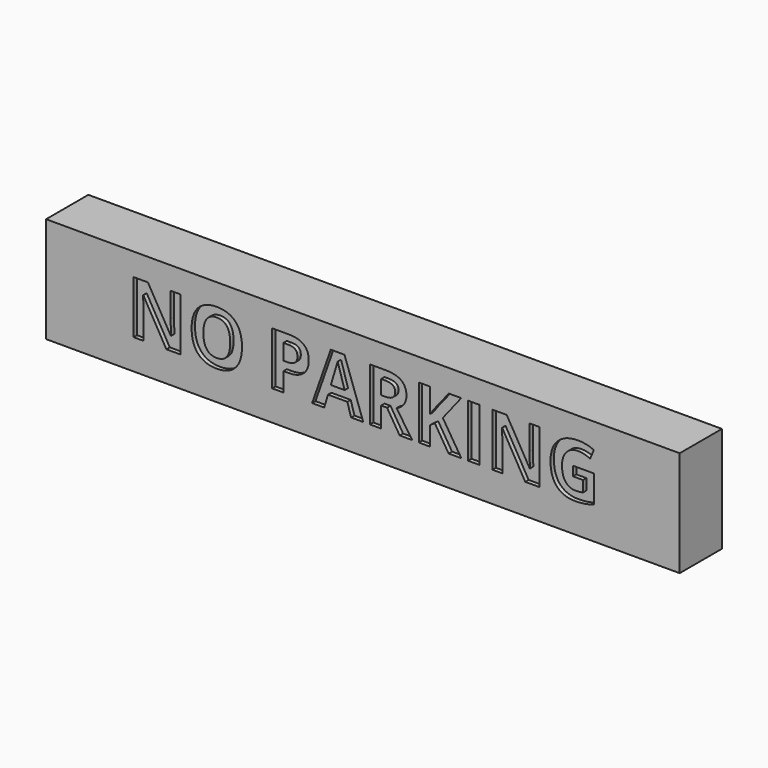
from build123d import *

# Parameters (mm, degrees)
F0_W         = 300
F0_H         = 50
F1_DEPTH     = 25
F2_TEXT_SIZE = 35.0935850292
F3_DEPTH     = 2


# Not quite as in the source:
# - Text() gives the source's letters only with a copy of the font that has no kerning and outlines rounded to 1/6400 em; it was checked with that copy


with BuildPart() as f1:
    # F0 (on Front) → F1 (new body)
    with BuildSketch(Plane.XZ):
        Rectangle(F0_W, F0_H)
    extrude(amount=F1_DEPTH)

    # F2 (on face) → F3 (cut)
    with BuildSketch(Plane.XZ.offset(25)):
        with Locations((-111.6661425513, -10.7)):
            Text('NO PARKING', F2_TEXT_SIZE, font='Open Sans', font_style=FontStyle.BOLD, text_align=(TextAlign.LEFT, TextAlign.BOTTOM))
    extrude(amount=-F3_DEPTH, mode=Mode.SUBTRACT)


solid = f1.part
